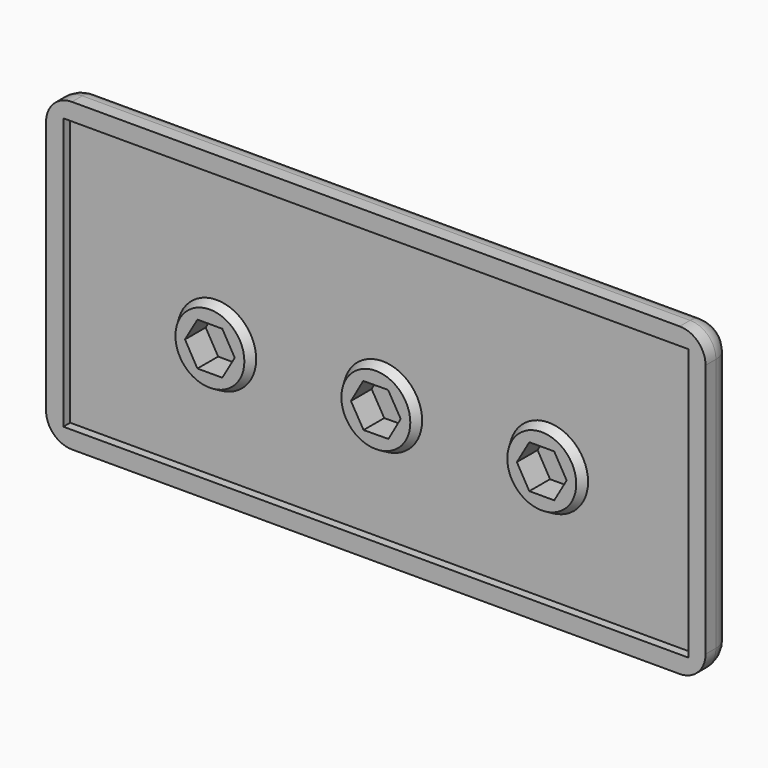
from build123d import *

# Parameters (mm, degrees)
F0_W          = 76.5
F0_H          = 35.5
F1_DEPTH      = 4
F2_W          = 72.5
F2_H          = 31.5
F3_DEPTH      = 1
F5_R          = 6
F7_DEPTH      = 1
F6_R          = 6
F8_DEPTH      = 1
F13_DEPTH     = 3
F14_R         = 2.5
F15_T1_DEPTH  = 11.5
F15_T4_ANGLE  = 90
F15_T6_ANGLE  = 90
F15_T8_ANGLE  = 90
F15_T10_ANGLE = 90


# Not quite as in the source:
# - a fillet or chamfer that OpenCascade refuses, or shapes differently, is made with other operations: its cross-section is extruded or revolved along the edge and cut away or added


with BuildPart() as f1:
    # F0 (on Front) → F1 (new body)
    with BuildSketch(Plane.XZ):
        Rectangle(F0_W, F0_H)
    extrude(amount=F1_DEPTH)

    # F2 (on face) → F3 (cut)
    with BuildSketch(Plane.XZ.offset(4)):
        Rectangle(F2_W, F2_H)
    extrude(amount=-F3_DEPTH, mode=Mode.SUBTRACT)

    # F5 (on face) → F7 (join)
    with BuildSketch(Plane.XZ.offset(3)):
        with Locations((0, -2.25)):
            Circle(F5_R)
    extrude(amount=F7_DEPTH)

    # F6 (on face) → F8 (join)
    with BuildSketch(Plane.XZ.offset(3)):
        with Locations((19.25, -2.25)):
            Circle(F6_R)
        with Locations((-19.25, -2.25)):
            Circle(F6_R)
    extrude(amount=F8_DEPTH)

    # F9: chamfer of 2 x 3.5 on 3 edges, made by hand


with BuildPart() as f9_tool2:
    # F9_s3 → F9_t4 (revolve)
    with BuildSketch(Plane.XY.offset(-2.25)):
        Polygon((6, -0.5), (4, -4), (6, -4), align=None)
    revolve(axis=Axis((0, -4, -2.25), (0, -1, 0)))

    split(bisect_by=Plane.XZ.offset(3), keep=Keep.TOP)


with BuildPart() as f1_1:
    add(f1.part)

    # F9_t1: cut F9_tool2
    add(f9_tool2.part, mode=Mode.SUBTRACT)


with BuildPart() as f9_tool7:
    # F9_s8 → F9_t9 (revolve)
    with BuildSketch(Plane.XY.offset(-2.25)):
        Polygon((-13.25, -0.5), (-15.25, -4), (-13.25, -4), align=None)
    revolve(axis=Axis((-19.25, -4, -2.25), (0, -1, 0)))

    split(bisect_by=Plane.XZ.offset(3), keep=Keep.TOP)


with BuildPart() as f1_2:
    add(f1_1.part)

    # F9_t6: cut F9_tool7
    add(f9_tool7.part, mode=Mode.SUBTRACT)


with BuildPart() as f9_tool12:
    # F9_s13 → F9_t14 (revolve)
    with BuildSketch(Plane.XY.offset(-2.25)):
        Polygon((25.25, -0.5), (23.25, -4), (25.25, -4), align=None)
    revolve(axis=Axis((19.25, -4, -2.25), (0, -1, 0)))

    split(bisect_by=Plane.XZ.offset(3), keep=Keep.TOP)


with BuildPart() as f1_3:
    add(f1_2.part)

    # F9_t11: cut F9_tool12
    add(f9_tool12.part, mode=Mode.SUBTRACT)

    # F10 (on face) + F12 (on face) + F11 (on face) → F13 (cut)
    with BuildSketch(Plane.XZ.offset(4)):
        Polygon((-1.464609527, 0.2376197995), (-2.8866467048, -2.2745791573), (-1.4220371778, -4.7621989567), (1.464609527, -4.7376197995), (2.8866467048, -2.2254208427), (1.4220371778, 0.2621989567), align=None)
    with BuildSketch(Plane.XZ.offset(4)):
        Polygon((-17.806624327, 0.25), (-20.693375673, 0.25), (-22.1367513459, -2.25), (-20.693375673, -4.75), (-17.806624327, -4.75), (-16.3632486541, -2.25), align=None)
    with BuildSketch(Plane.XZ.offset(4)):
        Polygon((20.693375673, 0.25), (17.806624327, 0.25), (16.3632486541, -2.25), (17.806624327, -4.75), (20.693375673, -4.75), (22.1367513459, -2.25), align=None)
    extrude(amount=-F13_DEPTH, mode=Mode.SUBTRACT)

    # F14
    f14_edges = [f1_3.edges().sort_by_distance(p)[0] for p in [
        (0, 0, 17.75),
        (38.25, 0, 0),
        (0, 0, -17.75),
        (-38.25, 0, 0),
    ]]
    fillet(f14_edges, radius=F14_R)

    # F15: fillet of radius 3 on 8 edges, made by hand

    # F15_s2 → F15_t1 (cut)
    with BuildSketch(Plane.XZ):
        with BuildLine():
            ThreePointArc((35.25, 17.75), (37.3713203436, 16.8713203436), (38.25, 14.75))
            Line((38.25, 14.75), (38.25, 17.75))
            Line((38.25, 17.75), (35.25, 17.75))
        make_face()
        with BuildLine():
            ThreePointArc((38.25, -14.75), (37.3713203436, -16.8713203436), (35.25, -17.75))
            Line((35.25, -17.75), (38.25, -17.75))
            Line((38.25, -17.75), (38.25, -14.75))
        make_face()
        with BuildLine():
            ThreePointArc((-35.25, 17.75), (-37.3713203436, 16.8713203436), (-38.25, 14.75))
            Line((-38.25, 14.75), (-38.25, 17.75))
            Line((-38.25, 17.75), (-35.25, 17.75))
        make_face()
        with BuildLine():
            ThreePointArc((-38.25, -14.75), (-37.3713203436, -16.8713203436), (-35.25, -17.75))
            Line((-35.25, -17.75), (-38.25, -17.75))
            Line((-38.25, -17.75), (-38.25, -14.75))
        make_face()
    extrude(amount=F15_T1_DEPTH, mode=Mode.SUBTRACT)

    # F15_s3 → F15_t4 (revolve, cut)
    with BuildSketch(Plane.YZ.offset(35.25)):
        with BuildLine():
            ThreePointArc((0, 15.25), (-0.732233047, 17.017766953), (-2.5, 17.75))
            Line((-2.5, 17.75), (0, 17.75))
            Line((0, 17.75), (0, 15.25))
        make_face()
    revolve(axis=Axis((35.25, 0, 14.75), (0, 1, 0)), revolution_arc=F15_T4_ANGLE, mode=Mode.SUBTRACT)

    # F15_s5 → F15_t6 (revolve, cut)
    with BuildSketch(Plane.XY.offset(-14.75)):
        with BuildLine():
            ThreePointArc((35.75, 0), (37.517766953, -0.732233047), (38.25, -2.5))
            Line((38.25, -2.5), (38.25, 0))
            Line((38.25, 0), (35.75, 0))
        make_face()
    revolve(axis=Axis((35.25, 0, -14.75), (0, 1, 0)), revolution_arc=F15_T6_ANGLE, mode=Mode.SUBTRACT)

    # F15_s7 → F15_t8 (revolve, cut)
    with BuildSketch(Plane.XY.offset(14.75)):
        with BuildLine():
            ThreePointArc((-35.75, 0), (-37.517766953, -0.732233047), (-38.25, -2.5))
            Line((-38.25, -2.5), (-38.25, 0))
            Line((-38.25, 0), (-35.75, 0))
        make_face()
    revolve(axis=Axis((-35.25, 0, 14.75), (0, 1, 0)), revolution_arc=F15_T8_ANGLE, mode=Mode.SUBTRACT)

    # F15_s9 → F15_t10 (revolve, cut)
    with BuildSketch(Plane.YZ.offset(-35.25)):
        with BuildLine():
            ThreePointArc((0, -15.25), (-0.732233047, -17.017766953), (-2.5, -17.75))
            Line((-2.5, -17.75), (0, -17.75))
            Line((0, -17.75), (0, -15.25))
        make_face()
    revolve(axis=Axis((-35.25, 0, -14.75), (0, 1, 0)), revolution_arc=F15_T10_ANGLE, mode=Mode.SUBTRACT)


solid = f1_3.part
